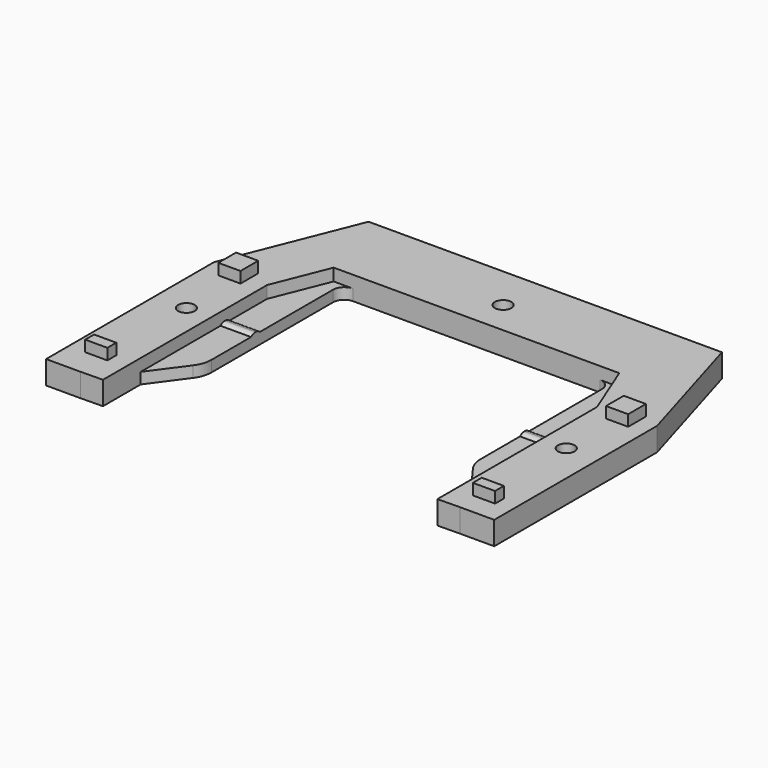
from build123d import *

# Parameters (mm, degrees)
F1_DEPTH      = 2
F2_DEPTH      = 4.2
F3_DEPTH      = 6.2
F4_DEPTH      = 6.2
F5_W          = 4
F5_H          = 2
F5_H_2        = 4
F6_DEPTH      = 2
F7_R          = 2.5
F7_R_2        = 1.5
F8_DEPTH      = 2.5
F9_DEPTH      = 4.5
F10_R         = 5
F12_START     = -1.7
F11_R         = 2.5
F11_R_2       = 1.5
F12_DEPTH     = 5.1
F13_DEPTH     = 4.2
F14_W         = 5.5
F14_H         = 2
F15_DEPTH     = 0.4
F16_T1_DEPTH  = 7.9494897428
F16_T3_DEPTH  = 7.9494897428
F17_S5_R      = 1.5
F17_T6_DEPTH  = 5
F17_S11_R     = 1.5
F17_T12_DEPTH = 5
F17_S17_R     = 1.5
F17_T18_DEPTH = 5


# Not quite as in the source:
# - a fillet or chamfer that OpenCascade refuses, or shapes differently, is made with other operations: its cross-section is extruded or revolved along the edge and cut away or added


with BuildPart() as f1:
    # F0 (on Top) → F1 (new body)
    with BuildSketch(Plane.XY):
        with BuildLine():
            Line((26, 14.25), (22.5, 14.25))
            ThreePointArc((22.5, 14.25), (23.9142135624, 13.6642135624), (24.5, 12.25))
            Line((24.5, 12.25), (24.5, -16.75))
            Line((24.5, -16.75), (30, -24.25))
            Line((30, -24.25), (30, 4.25))
            Line((30, 4.25), (26, 14.25))
        make_face()
    extrude(amount=F1_DEPTH)



with BuildPart() as f1b:
    # F0 (on Top) → F1, piece 2 (new body)
    with BuildSketch(Plane.XY):
        with BuildLine():
            Line((-22, 14.25), (-25.5, 14.25))
            Line((-25.5, 14.25), (-29.5, 4.25))
            Line((-29.5, 4.25), (-29.5, -24.25))
            Line((-29.5, -24.25), (-24, -16.75))
            Line((-24, -16.75), (-24, 12.25))
            ThreePointArc((-24, 12.25), (-23.4142135624, 13.6642135624), (-22, 14.25))
        make_face()
    extrude(amount=F1_DEPTH)


with BuildPart() as f1_1:
    add(f1.part)

    add(f1b.part)  # F2 merges F1b
    # F0 (on Top) → F2 (join)
    with BuildSketch(Plane.XY):
        Polygon((-29.5, 4.25), (-25.5, 14.25), (-22, 14.25), (22.5, 14.25), (26, 14.25), (30, 4.25), (30, -24.25), (30, -31.75), (34, -31.6827731092), (34, 5.0203296143), (27.1081318457, 28.25), (-24.2081318457, 28.25), (-33.5, 5.0203296143), (-33.5, -32.8172268908), (-29.5, -32.75), (-29.5, -24.25), align=None)
    extrude(amount=F2_DEPTH)

    # F3 (add): faces of the model
    f3_faces = [f1_1.faces().sort_by_distance(p)[0] for p in [
        (-33.5, -13.8984486382, 2.1),
        (-28.8540659229, 16.6351648071, 2.1),
    ]]
    extrude(f3_faces, amount=F3_DEPTH, dir=(-1, 0, 0))

    # F4 (add): faces of the model
    f4_faces = [f1_1.faces().sort_by_distance(p)[0] for p in [
        (34, -13.3312217475, 2.1),
        (30.5540659229, 16.6351648071, 2.1),
    ]]
    extrude(f4_faces, amount=F4_DEPTH, dir=(1, 0, 0))

    # F5 (on face) → F6 (join)
    with BuildSketch(Plane.XY.offset(4.2)):
        with Locations((-34.7, -26.75)):
            Rectangle(F5_W, F5_H)
        with Locations((35.2, -26.75)):
            Rectangle(F5_W, F5_H)
        with Locations((35.2, 4.25)):
            Rectangle(F5_W, F5_H_2)
        with Locations((-34.7, 4.25)):
            Rectangle(F5_W, F5_H_2)
    extrude(amount=F6_DEPTH)

    # F7 (on face) → F8 (cut)
    with BuildSketch(Plane(origin=(0, 0, 0), x_dir=(1, 0, 0), z_dir=(0, 0, -1))):
        with Locations((-34, 8.3172268908)):
            Circle(F7_R)
        with Locations((-34, 8.3172268908)):
            Circle(F7_R_2, mode=Mode.SUBTRACT)
        with Locations((34.5, 8.3172268908)):
            Circle(F7_R)
        with Locations((34.5, 8.3172268908)):
            Circle(F7_R_2, mode=Mode.SUBTRACT)
    extrude(amount=-F8_DEPTH, mode=Mode.SUBTRACT)

    # F9 (cut): faces of the model
    f9_faces = [f1_1.faces().sort_by_distance(p)[0] for p in [
        (-34, -8.3172268908, 0),
        (34.5, -8.3172268908, 0),
    ]]
    extrude(f9_faces, amount=-F9_DEPTH, mode=Mode.SUBTRACT)

    # F10
    f10_edges = [f1_1.edges().sort_by_distance(p)[0] for p in [
        (24.5, -16.75, 1),
        (-24, -16.75, 1),
    ]]
    fillet(f10_edges, radius=F10_R)

    # F11 (on face) → F12 (cut)
    with BuildSketch(Plane.XY.offset(4.2).offset(F12_START)):
        with Locations((0.25, 20.25)):
            Circle(F11_R)
        with Locations((0.25, 20.25)):
            Circle(F11_R_2, mode=Mode.SUBTRACT)
    extrude(amount=-F12_DEPTH, mode=Mode.SUBTRACT)

    # F11 (on face) → F13 (cut)
    with BuildSketch(Plane.XY.offset(4.2)):
        with Locations((0.25, 20.25)):
            Circle(F11_R_2)
    extrude(amount=-F13_DEPTH, mode=Mode.SUBTRACT)

    # F14 (on face) → F15 (join)
    with BuildSketch(Plane.XY.offset(2)):
        with Locations((27.25, -5.25)):
            Rectangle(F14_W, F14_H)
        with Locations((-26.75, -5.25)):
            Rectangle(F14_W, F14_H)
    extrude(amount=F15_DEPTH)

    # F16: fillet of radius 1.4 on 4 edges, made by hand

    # F16_s2 → F16_t1 (cut)
    with BuildSketch(Plane.YZ.offset(-29.5)):
        with BuildLine():
            ThreePointArc((-6.25, 2), (-5.7993543651, 2.2961481397), (-5.2702041029, 2.4))
            Line((-5.2702041029, 2.4), (-6.25, 2.4))
            Line((-6.25, 2.4), (-6.25, 2))
        make_face()
        with BuildLine():
            ThreePointArc((-5.2297958971, 2.4), (-4.7006456349, 2.2961481397), (-4.25, 2))
            Line((-4.25, 2), (-4.25, 2.4))
            Line((-4.25, 2.4), (-5.2297958971, 2.4))
        make_face()
    extrude(amount=F16_T1_DEPTH, mode=Mode.SUBTRACT)

    # F16_s4 → F16_t3 (cut)
    with BuildSketch(Plane.YZ.offset(22.0505102572)):
        with BuildLine():
            ThreePointArc((-4.25, 2), (-4.7006456349, 2.2961481397), (-5.2297958971, 2.4))
            Line((-5.2297958971, 2.4), (-4.25, 2.4))
            Line((-4.25, 2.4), (-4.25, 2))
        make_face()
        with BuildLine():
            ThreePointArc((-5.2702041029, 2.4), (-5.7993543651, 2.2961481397), (-6.25, 2))
            Line((-6.25, 2), (-6.25, 2.4))
            Line((-6.25, 2.4), (-5.2702041029, 2.4))
        make_face()
    extrude(amount=F16_T3_DEPTH, mode=Mode.SUBTRACT)

    # F17: chamfer of 1.2 on 3 edges, made by hand


with BuildPart() as f17_tool2:
    # F17_s3 → F17_t4 (revolve)
    with BuildSketch(Plane.XZ.offset(8.3172268908)):
        Polygon((-31.5, 1.3), (-32.7, 2.5), (-31.5, 2.5), align=None)
    revolve(axis=Axis((-34, -8.3172268908, 2.5), (0, 0, -1)))

    # F17_s5 → F17_t6 (cut, symmetric)
    with BuildSketch(Plane.XY.offset(1.9)):
        with Locations((-34, -8.3172268908)):
            Circle(F17_S5_R)
    extrude(amount=F17_T6_DEPTH, both=True, mode=Mode.SUBTRACT)


with BuildPart() as f1_2:
    add(f1_1.part)

    # F17_t1: union F17_tool2
    add(f17_tool2.part)


with BuildPart() as f17_tool8:
    # F17_s9 → F17_t10 (revolve)
    with BuildSketch(Plane.XZ.offset(8.3172268908)):
        Polygon((37, 1.3), (35.8, 2.5), (37, 2.5), align=None)
    revolve(axis=Axis((34.5, -8.3172268908, 2.5), (0, 0, -1)))

    # F17_s11 → F17_t12 (cut, symmetric)
    with BuildSketch(Plane.XY.offset(1.9)):
        with Locations((34.5, -8.3172268908)):
            Circle(F17_S11_R)
    extrude(amount=F17_T12_DEPTH, both=True, mode=Mode.SUBTRACT)


with BuildPart() as f1_3:
    add(f1_2.part)

    # F17_t7: union F17_tool8
    add(f17_tool8.part)


with BuildPart() as f17_tool14:
    # F17_s15 → F17_t16 (revolve)
    with BuildSketch(Plane.XZ.offset(-20.25)):
        Polygon((2.75, 1.3), (1.55, 2.5), (2.75, 2.5), align=None)
    revolve(axis=Axis((0.25, 20.25, 2.5), (0, 0, 1)))

    # F17_s17 → F17_t18 (cut, symmetric)
    with BuildSketch(Plane.XY.offset(1.9)):
        with Locations((0.25, 20.25)):
            Circle(F17_S17_R)
    extrude(amount=F17_T18_DEPTH, both=True, mode=Mode.SUBTRACT)


with BuildPart() as f1_4:
    add(f1_3.part)

    # F17_t13: union F17_tool14
    add(f17_tool14.part)


solid = f1_4.part
